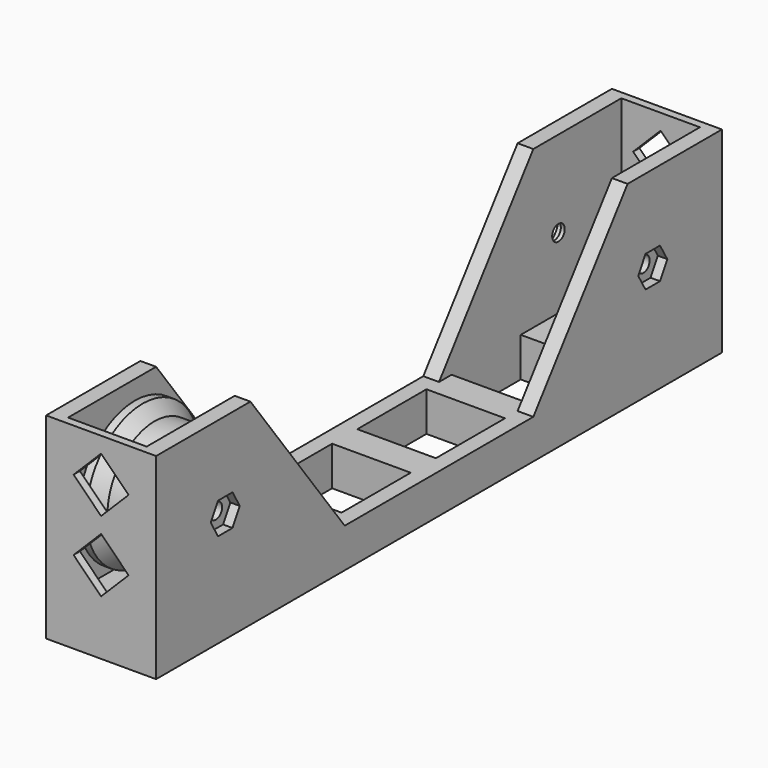
from build123d import *

# Parameters (mm, degrees)
F0_R      = 15
F1_DEPTH  = 14
F2_W      = 20
F2_H      = 30
F3_DEPTH  = 40
F2_H_2    = 58
F2_H_3    = 28
F4_DEPTH  = 40
F9_D      = 4
F9_2_D    = 4
F10_W     = 20
F10_H     = 22
F11_DEPTH = 10
F12_DEPTH = 2.4
F13_R     = 5
F14_DEPTH = 3
F16_DEPTH = 180.001


with BuildPart() as f1:
    # F0 (on Right) → F1 (new body, symmetric)
    with BuildSketch(Plane.YZ):
        Polygon((-90, 0), (0, 0), (90, 0), (90, 50), (60, 50), (30, 10), (0, 10), (-30, 10), (-60, 50), (-90, 50), align=None)
        with Locations((-68, 28)):
            Circle(F0_R, mode=Mode.SUBTRACT)
        with Locations((-68, 28)):
            Circle(F0_R)
    extrude(amount=F1_DEPTH, both=True)

    # F2 (on face) → F3 (cut, through all)
    with BuildSketch(Plane.XY.offset(50)):
        with Locations((0, -45)):
            Rectangle(F2_W, F2_H)
    extrude(amount=-F3_DEPTH, mode=Mode.SUBTRACT)

    # F2 (on face) → F4 (cut, through all)
    with BuildSketch(Plane.XY.offset(50)):
        with Locations((0, 59)):
            Rectangle(F2_W, F2_H_2)
        with Locations((0, -74)):
            Rectangle(F2_W, F2_H_3)
    extrude(amount=-F4_DEPTH, mode=Mode.SUBTRACT)

    # F9 (through all)
    with Locations(Plane.YZ.offset(14)):
        with Locations((-68, 28), (68, 28)):
            Hole(F9_D / 2)

    # F10 (on face) → F11 (cut, through all)
    with BuildSketch(Plane.XY.offset(10)):
        with Locations((0, 15)):
            Rectangle(F10_W, F10_H)
        with Locations((0, -15)):
            Rectangle(F10_W, F10_H)
        with Locations((0, -45)):
            Rectangle(F10_W, F10_H)
        with Locations((0, 45)):
            Rectangle(F10_W, F10_H)
    extrude(amount=-F11_DEPTH, mode=Mode.SUBTRACT)

    # F8 (on face) → F12 (cut, through all)
    with BuildSketch(Plane.YZ.offset(14)):
        Polygon((-70.3094010768, 24), (-65.6905989232, 24), (-63.3811978465, 28), (-65.6905989232, 32), (-70.3094010768, 32), (-72.6188021535, 28), align=None)
        Polygon((70.3094010768, 32), (65.6905989232, 32), (63.3811978465, 28), (65.6905989232, 24), (70.3094010768, 24), (72.6188021535, 28), align=None)
    extrude(amount=-F12_DEPTH, mode=Mode.SUBTRACT)

    # F13 (on face) → F14 (cut)
    with BuildSketch(Plane(origin=(-14, 0, 0), x_dir=(0, -1, 0), z_dir=(-1, 0, 0))):
        with Locations((68, 28)):
            Circle(F13_R)
        with Locations((-68, 28)):
            Circle(F13_R)
    extrude(amount=-F14_DEPTH, mode=Mode.SUBTRACT)

    # F15 (on face) → F16 (cut, through all)
    with BuildSketch(Plane(origin=(0, 90, 0), x_dir=(-1, 0, 0), z_dir=(0, 1, 0))):
        Polygon((-7, 39), (0, 32), (7, 39), (0, 46), align=None)
        Polygon((7, 21), (0, 28), (-7, 21), (0, 14), align=None)
    extrude(amount=-F16_DEPTH, mode=Mode.SUBTRACT)


with BuildPart() as f7:
    # F6 (on plane+point) → F7 (revolve)
    with BuildSketch(Plane.XZ.offset(68)):
        Polygon((4, 43), (0, 43), (-4, 43), (-7, 46), (-9, 46), (-9, 28), (0, 28), (9, 28), (9, 46), (7, 46), align=None)
    revolve(axis=Axis((-4.5, -68, 28), (1, 0, 0)))

    # F9#2 (through all)
    with Locations(Plane.YZ.offset(14)):
        with Locations((-68, 28), (68, 28)):
            Hole(F9_2_D / 2)


solid = Compound([f1.part, f7.part])
